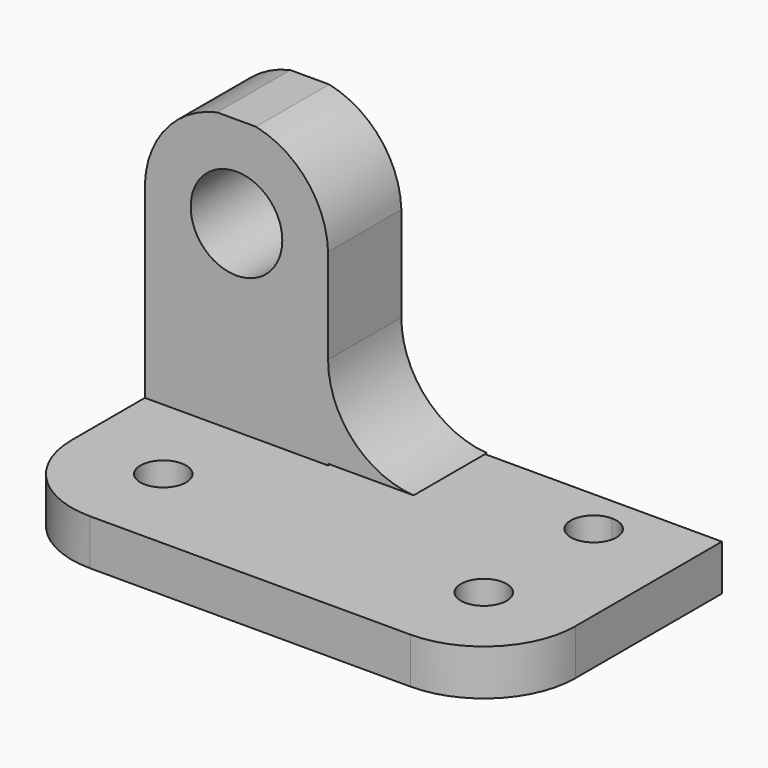
from build123d import *

# Parameters (mm, degrees)
F1_DEPTH  = 38.1
F2_W      = 25.4
F2_H      = 38.1
F3_DEPTH  = 25.4
F4_R      = 6.35
F5_DEPTH  = 12.701
F7_DEPTH  = 12.701
F8_W      = 12.7
F8_H      = 12.7
F9_DEPTH  = 12.7
F11_DEPTH = 12.701
F13_DEPTH = 6.351
F14_R     = 3.175
F15_DEPTH = 6.351


with BuildPart() as f1:
    # F0 (on Front) → F1 (new body)
    with BuildSketch(Plane.XZ):
        Polygon((25.4, 44.45), (0, 44.45), (0, 0), (69.85, 0), (69.85, 6.35), (25.4, 6.35), align=None)
    extrude(amount=F1_DEPTH)

    # F2 (on face) → F3 (cut)
    with BuildSketch(Plane.XZ.offset(38.1)):
        with Locations((12.7, 25.4)):
            Rectangle(F2_W, F2_H)
    extrude(amount=-F3_DEPTH, mode=Mode.SUBTRACT)

    # F4 (on face) → F5 (cut, through all)
    with BuildSketch(Plane.XZ.offset(12.7)):
        with Locations((12.7, 31.75)):
            Circle(F4_R)
    extrude(amount=-F5_DEPTH, mode=Mode.SUBTRACT)

    # F6 (on face) → F7 (cut, through all)
    with BuildSketch(Plane.XZ.offset(12.7)):
        with BuildLine():
            ThreePointArc((0, 32.429072573), (-0.0062022328, 32.0321151685), (0, 31.635157764))
            Line((0, 31.635157764), (0, 32.429072573))
        make_face()
        with BuildLine():
            ThreePointArc((19.05, 31.75), (12.642576534, 38.0997403526), (6.3510385683, 31.635157764))
            Line((6.3510385683, 31.635157764), (19.0489614317, 31.635157764))
            ThreePointArc((19.0489614317, 31.635157764), (19.0497403526, 31.692576534), (19.05, 31.75))
        make_face()
        with BuildLine():
            Line((0, 44.45), (0, 32.429072573))
            ThreePointArc((0, 32.429072573), (2.9352888733, 40.1621823142), (10.0085855964, 44.45))
            Line((10.0085855964, 44.45), (0, 44.45))
        make_face()
        with BuildLine():
            ThreePointArc((15.3914144036, 44.45), (12.7, 44.7383174013), (10.0085855964, 44.45))
            Line((10.0085855964, 44.45), (15.3914144036, 44.45))
        make_face()
        with BuildLine():
            Line((25.4, 32.429072573), (25.4, 31.635157764))
            ThreePointArc((25.4, 31.635157764), (25.4062022328, 32.0321151685), (25.4, 32.429072573))
        make_face()
        with BuildLine():
            Line((25.4, 44.45), (15.3914144036, 44.45))
            ThreePointArc((15.3914144036, 44.45), (22.4647111267, 40.1621823142), (25.4, 32.429072573))
            Line((25.4, 32.429072573), (25.4, 44.45))
        make_face()
    extrude(amount=-F7_DEPTH, mode=Mode.SUBTRACT)

    # F8 (on Front) → F9 (join)
    with BuildSketch(Plane.XZ):
        with Locations((30.9091203046, 12.9094149452)):
            Rectangle(F8_W, F8_H)
    extrude(amount=F9_DEPTH)

    # F10 (on face) → F11 (cut, through all)
    with BuildSketch(Plane.XZ.offset(12.7)):
        with BuildLine():
            Line((37.2591203046, 19.2594149452), (25.4, 19.2594149452))
            ThreePointArc((25.4, 19.2594149452), (28.8257307878, 10.5713666258), (37.2591203046, 6.5594149452))
            Line((37.2591203046, 6.5594149452), (37.2591203046, 19.2594149452))
        make_face()
    extrude(amount=-F11_DEPTH, mode=Mode.SUBTRACT)

    # F12 (on face) → F13 (cut, through all)
    with BuildSketch(Plane.XY.offset(6.35)):
        with BuildLine():
            ThreePointArc((12.7, -38.1), (3.7197438789, -34.3802561211), (0, -25.4))
            Line((0, -25.4), (0, -38.1))
            Line((0, -38.1), (12.7, -38.1))
        make_face()
        with BuildLine():
            ThreePointArc((69.85, -25.4), (66.1302561211, -34.3802561211), (57.15, -38.1))
            Line((57.15, -38.1), (69.85, -38.1))
            Line((69.85, -38.1), (69.85, -25.4))
        make_face()
    extrude(amount=-F13_DEPTH, mode=Mode.SUBTRACT)

    # F14 (on face) → F15 (cut, through all)
    with BuildSketch(Plane.XY.offset(6.35)):
        with BuildLine():
            ThreePointArc((15.875, -25.4), (12.7, -22.225), (9.525, -25.4))
            ThreePointArc((9.525, -25.4), (12.7, -28.575), (15.875, -25.4))
        make_face()
        with Locations((57.15, -25.4)):
            Circle(F14_R)
        with BuildLine():
            Line((57.15, -9.525), (57.15, -3.175))
            ThreePointArc((57.15, -3.175), (53.975, -6.35), (57.15, -9.525))
        make_face()
        with BuildLine():
            ThreePointArc((60.325, -6.35), (59.3950640303, -4.1049359697), (57.15, -3.175))
            Line((57.15, -3.175), (57.15, -9.525))
            ThreePointArc((57.15, -9.525), (59.3950640303, -8.5950640303), (60.325, -6.35))
        make_face()
    extrude(amount=-F15_DEPTH, mode=Mode.SUBTRACT)


solid = f1.part
